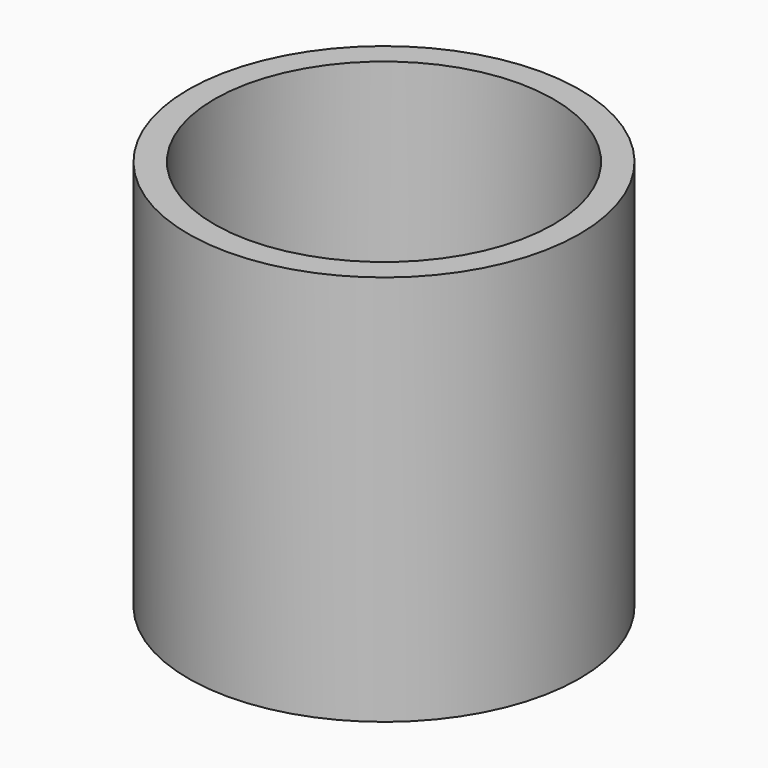
from build123d import *

# Parameters (mm, degrees)
F0_R     = 9.525
F1_DEPTH = 19.05
F2_T     = -1.27
F4_D     = 0.635


# Not quite as in the source:
# - the program builds the solid bodies; features that only make, move or delete a surface that nothing else refers to are left out


with BuildPart() as f1:
    # F0 (on Top) → F1 (new body)
    with BuildSketch(Plane.XY):
        with Locations((-115.1416823268, 52.6224188507)):
            Circle(F0_R)
    extrude(amount=F1_DEPTH)

    # F2
    f2_openings = [f1.faces().sort_by_distance(p)[0] for p in [
        (-115.141682, 52.622419, 19.05),
    ]]
    offset(amount=F2_T, openings=f2_openings)

    # F4 (through all)
    with Locations(Plane.XY.offset(1.27)):
        with Locations((-116.9411316514, 59.9756650627), (-114.9873510003, 58.9685030282), (-113.8059347868, 58.9685030282), (-117.4980401993, 58.4304407239), (-119.3492934108, 57.1395158768), (-121.0996806622, 55.9318587184), (-119.9708729982, 54.7268129885), (-116.9627532363, 57.0406801999), (-116.2916645408, 56.6788762808), (-117.056325078, 55.0978146493), (-118.0468276143, 53.8730248809), (-120.9187433124, 52.0108155906), (-120.5618828535, 51.0843060911), (-118.0632561445, 51.9599355757), (-118.6012327671, 48.8700121641), (-117.4913495779, 49.2096692324), (-115.4741570354, 50.8750453591), (-115.1792779565, 53.5607412457), (-114.4042313099, 57.1855939925), (-113.5956719518, 55.5465482175), (-111.127205193, 57.0756867528), (-110.8181774616, 56.6184930503), (-112.3543679714, 54.7396689653), (-111.7949485779, 52.8271049261), (-110.0980043411, 54.0584772825), (-110.5114147067, 51.1053167284), (-113.6578395963, 51.2212850153), (-114.1850054264, 49.5988503098), (-112.0592430234, 48.9115975797), (-115.2876019478, 47.3995991051), (-112.5525608659, 57.9002201557)):
            Hole(F4_D / 2)


solid = f1.part
